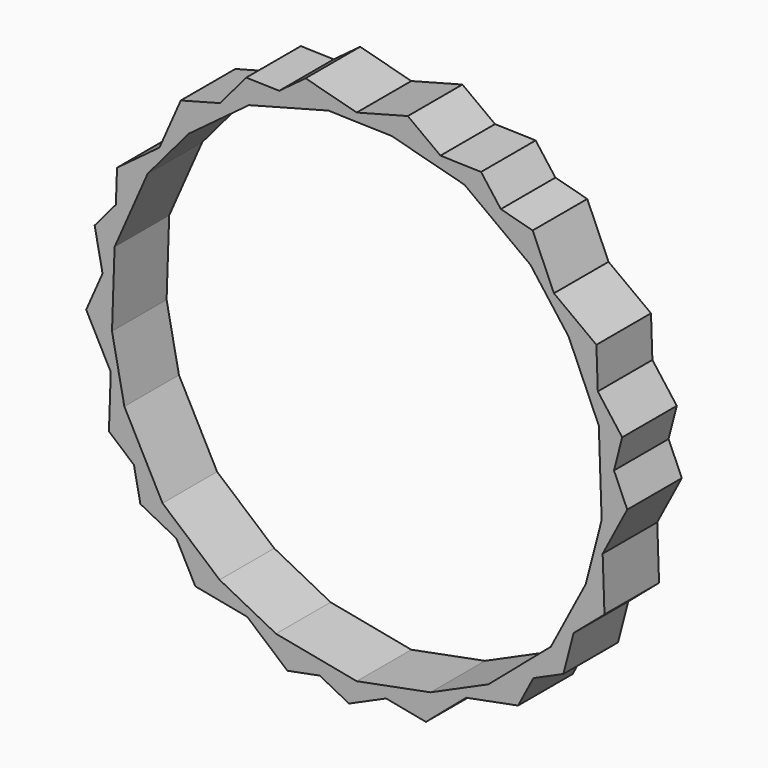
from build123d import *

# Parameters (mm, degrees)
F1_DEPTH = 12.7


with BuildPart() as f1:
    # F0 (on Front) → F1 (new body)
    with BuildSketch(Plane.XZ):
        Polygon((36.7118305086, 29.2767078878), (32.7487252653, 38.2864065468), (26.8258066759, 39.8544200468), (32.3351986213, 32.527134341), align=None)
        Polygon((44.6137633316, 23.4081194068), (36.7118305086, 29.2767078878), (39.4362804042, 23.0829605448), (44.8738240342, 15.8512304175), align=None)
        Polygon((39.4362804042, 23.0829605448), (36.7118305086, 29.2767078878), (32.3351986213, 32.527134341), align=None)
        Polygon((32.3351986213, 32.527134341), (26.8258066759, 39.8544200468), (20.0559669896, 41.6466445828), align=None)
        Polygon((20.0559669896, 41.6466445828), (26.8258066759, 39.8544200468), (23.143676418, 44.7515158919), (15.5853806795, 44.9668488809), align=None)
        Polygon((44.8738240342, 15.8512304175), (39.4362804042, 23.0829605448), (45.0653487584, 10.2858717752), align=None)
        Polygon((6.5411333928, 45.2245160678), (20.0559669896, 41.6466445828), (15.5853806795, 44.9668488809), align=None)
        Polygon((44.8738240342, 15.8512304175), (45.0653487584, 10.2858717752), (47.8850571971, 3.8755642564), (49.4179902366, 9.8076589327), align=None)
        Polygon((47.8850571971, 3.8755642564), (45.0653487584, 10.2858717752), (45.5914042437, -5.0003397286), align=None)
        Polygon((-5.2700710808, 45.5610128193), (6.5411333928, 45.2245160678), (0, 46.9561936707), align=None)
        Polygon((0, 46.9561936707), (6.5411333928, 45.2245160678), (15.5853806795, 44.9668488809), (9.5150217621, 49.4751684548), align=None)
        Polygon((50.3520142156, -1.7328003913), (47.8850571971, 3.8755642564), (45.5914042437, -5.0003397286), (45.7789038594, -10.4487360706), align=None)
        Polygon((45.7789038594, -10.4487360706), (45.5914042437, -5.0003397286), (42.6351039178, -16.440535075), align=None)
        Polygon((-5.2700710808, 45.5610128193), (0, 46.9561936707), (-9.5150217621, 49.4751684548), (-14.433823419, 45.82208466), align=None)
        Polygon((-20.0559669896, 41.6466445828), (-5.2700710808, 45.5610128193), (-14.433823419, 45.82208466), align=None)
        Polygon((46.1174311574, -20.2857209931), (45.7789038594, -10.4487360706), (42.6351039178, -16.440535075), (40.371362632, -25.2006878565), align=None)
        Polygon((40.371362632, -25.2006878565), (42.6351039178, -16.440535075), (36.1396037465, -28.8203722726), align=None)
        Polygon((-25.4391722107, 40.2215129805), (-20.0559669896, 41.6466445828), (-14.433823419, 45.82208466), (-20.5582977883, 45.99656862), align=None)
        Polygon((-31.2796204782, 33.3110885798), (-20.0559669896, 41.6466445828), (-25.4391722107, 40.2215129805), align=None)
        Polygon((40.371362632, -25.2006878565), (36.1396037465, -28.8203722726), (32.8858829718, -35.0216704662), (38.4795494638, -32.5215652427), align=None)
        Polygon((32.8858829718, -35.0216704662), (36.1396037465, -28.8203722726), (24.5163525755, -38.7624559943), align=None)
        Polygon((-38.9068697692, 24.2865193693), (-31.2796204782, 33.3110885798), (-36.7118305086, 29.2767078878), align=None)
        Polygon((-36.7118305086, 29.2767078878), (-31.2796204782, 33.3110885798), (-25.4391722107, 40.2215129805), (-32.7487252653, 38.2864065468), align=None)
        Polygon((30.0392094677, -40.4471732921), (32.8858829718, -35.0216704662), (24.5163525755, -38.7624559943), (20.3735288846, -42.3060686525), align=None)
        Polygon((20.3735288846, -42.3060686525), (24.5163525755, -38.7624559943), (13.7288245836, -43.5839724576), align=None)
        Polygon((-38.9068697692, 24.2865193693), (-36.7118305086, 29.2767078878), (-44.6137633316, 23.4081194068), (-44.8244900831, 17.284784924), align=None)
        Polygon((-45.0653487584, 10.2858717752), (-38.9068697692, 24.2865193693), (-44.8244900831, 17.284784924), align=None)
        Polygon((12.8937326976, -48.703999732), (20.3735288846, -42.3060686525), (13.7288245836, -43.5839724576), (5.4684417421, -47.2759741742), align=None)
        Polygon((5.4684417421, -47.2759741742), (13.7288245836, -43.5839724576), (0, -46.2242881707), align=None)
        Polygon((-47.3075095617, 5.1885574364), (-45.0653487584, 10.2858717752), (-44.8244900831, 17.284784924), (-48.7794544472, 12.6052670182), align=None)
        Polygon((-45.5461821411, -3.6862680312), (-45.0653487584, 10.2858717752), (-47.3075095617, 5.1885574364), align=None)
        Polygon((5.4684417421, -47.2759741742), (0, -46.2242881707), (-6.8770318811, -47.5468730158), (-1.4347768951, -50.3613874713), align=None)
        Polygon((-6.8770318811, -47.5468730158), (0, -46.2242881707), (-15.0200126245, -43.3356522862), align=None)
        Polygon((-43.2460019659, -15.2762185204), (-45.5461821411, -3.6862680312), (-45.7789038594, -10.4487360706), align=None)
        Polygon((-45.7789038594, -10.4487360706), (-45.5461821411, -3.6862680312), (-47.3075095617, 5.1885574364), (-50.3520142156, -1.7328003913), align=None)
        Polygon((-12.8937326976, -48.703999732), (-6.8770318811, -47.5468730158), (-15.0200126245, -43.3356522862), (-20.3735288846, -42.3060686525), align=None)
        Polygon((-20.3735288846, -42.3060686525), (-15.0200126245, -43.3356522862), (-25.515539679, -37.9077896286), align=None)
        Polygon((-43.2460019659, -15.2762185204), (-45.7789038594, -10.4487360706), (-46.1174311574, -20.2857209931), (-41.4614014616, -24.2683104051), align=None)
        Polygon((-36.1396037465, -28.8203722726), (-43.2460019659, -15.2762185204), (-41.4614014616, -24.2683104051), align=None)
        Polygon((-30.0392094677, -40.4471732921), (-20.3735288846, -42.3060686525), (-25.515539679, -37.9077896286), (-33.5523273154, -33.7514876846), align=None)
        Polygon((-33.5523273154, -33.7514876846), (-25.515539679, -37.9077896286), (-36.1396037465, -28.8203722726), align=None)
        Polygon((-33.5523273154, -33.7514876846), (-36.1396037465, -28.8203722726), (-41.4614014616, -24.2683104051), (-40.2686869878, -30.2780577489), align=None)
    extrude(amount=F1_DEPTH)


solid = f1.part
